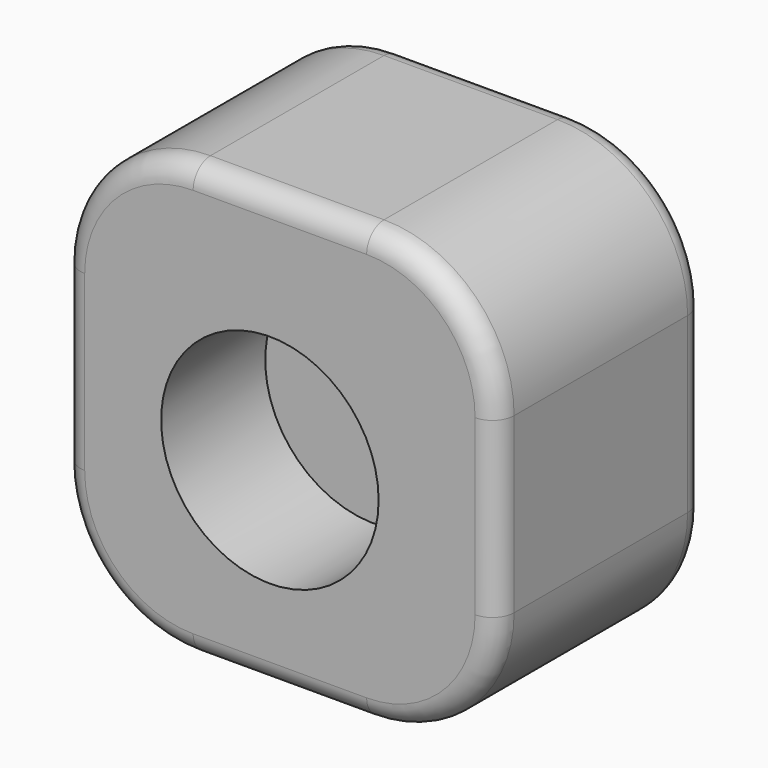
from build123d import *

# Parameters (mm, degrees)
F1_DEPTH = 60
F2_R     = 5
F3_R     = 25.0723290406
F4_DEPTH = 30


# Not quite as in the source:
# - a feature names something its author has since deleted; it is built from what else it names


with BuildPart() as f1:
    # F0 (on Front) → F1 (new body)
    with BuildSketch(Plane.XZ):
        with BuildLine():
            Line((21.3254676014, 72.3460770576), (-18.6745323986, 72.3460770576))
            ThreePointArc((-18.6745323986, 72.3460770576), (-39.8877358342, 63.5592804932), (-48.6745323986, 42.3460770576))
            Line((-48.6745323986, 42.3460770576), (-48.6745323986, 2.3460770576))
            ThreePointArc((-48.6745323986, 2.3460770576), (-39.8877358342, -18.867126378), (-18.6745323986, -27.6539229424))
            Line((-18.6745323986, -27.6539229424), (21.3254676014, -27.6539229424))
            ThreePointArc((21.3254676014, -27.6539229424), (42.538671037, -18.867126378), (51.3254676014, 2.3460770576))
            Line((51.3254676014, 2.3460770576), (51.3254676014, 42.3460770576))
            ThreePointArc((51.3254676014, 42.3460770576), (42.538671037, 63.5592804932), (21.3254676014, 72.3460770576))
        make_face()
    extrude(amount=F1_DEPTH)

    # F2
    f2_edges = [f1.edges().sort_by_distance(p)[0] for p in [
        (51.325468, -30, 42.346077),
        (21.325468, -30, 72.346077),
        (42.538671, 0, 63.55928),
        (42.538671, -60, 63.55928),
    ]]
    fillet(f2_edges, radius=F2_R)

    # F3 (on face) → F4 (cut)
    with BuildSketch(Plane.XZ.offset(60)):
        with Locations((-0.98494126, 18.3436237276)):
            Circle(F3_R)
    extrude(amount=-F4_DEPTH, mode=Mode.SUBTRACT)


solid = f1.part
